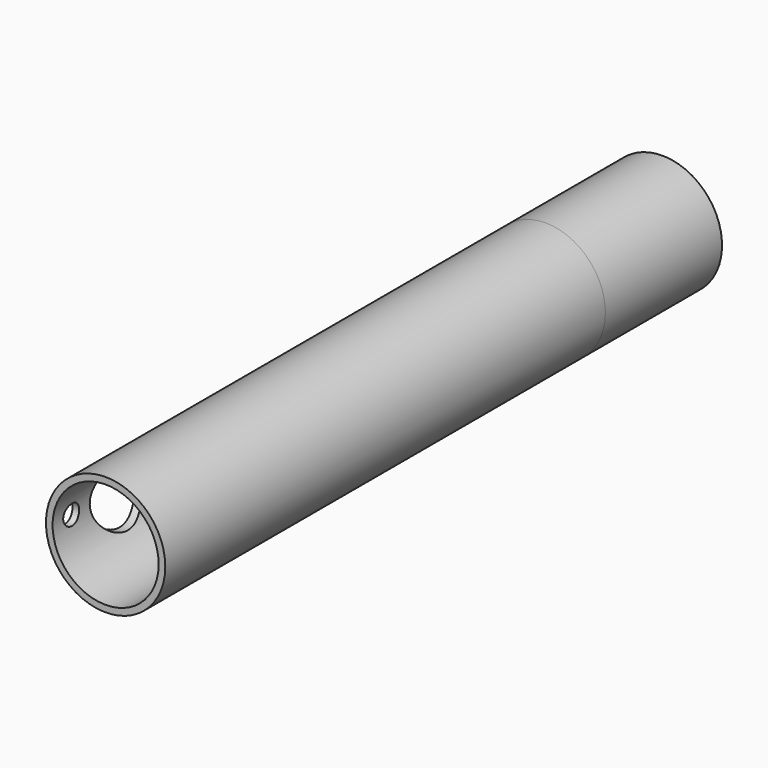
from build123d import *

# Parameters (mm, degrees)
F3_R      = 4.5
F4_DEPTH  = 32.5
F8_DEPTH  = 32.5
F6_R      = 4.5
F6_R_2    = 4
F9_DEPTH  = 9
F7_R      = 4.5
F7_R_2    = 4
F10_DEPTH = 11
F11_R     = 2.5
F11_R_2   = 0.75
F12_DEPTH = 4.501


# Not quite as in the source:
# - ends of sketch curves that miss each other by under 0.0002 mm in the source are joined


with BuildPart() as f4:
    # F3 (on Front) → F4 (new body)
    with BuildSketch(Plane.XZ):
        Circle(F3_R)
    extrude(amount=F4_DEPTH)

    # F5 (on face) → F8 (cut, through all)
    with BuildSketch(Plane.XZ.offset(32.5)):
        with BuildLine():
            Line((-1.25, -3.8), (0, -3.8))
            Line((0, -3.8), (1.25, -3.8))
            Line((1.25, -3.8), (1.25, -3.7))
            ThreePointArc((1.25, -3.7), (1.3085786438, -3.5585786438), (1.45, -3.5))
            Line((1.45, -3.5), (2, -3.5))
            Line((2, -3.5), (2, -3.05))
            ThreePointArc((2, -3.05), (2.0585786438, -2.9085786438), (2.2, -2.85))
            Line((2.2, -2.85), (3.15, -2.85))
            Line((3.15, -2.85), (3.15, -2.15))
            Line((3.15, -2.15), (2.2, -2.15))
            ThreePointArc((2.2, -2.15), (2.0585786438, -2.0914213562), (2, -1.95))
            Line((2, -1.95), (2, -1.887459))
            ThreePointArc((2, -1.887459), (2.1033535752, -1.771554046), (2.2, -1.65))
            Line((2.2, -1.65), (3.75, -1.65))
            Line((3.75, -1.65), (3.75, 0))
            Line((3.75, 0), (3.75, 1.65))
            Line((3.75, 1.65), (2.2, 1.65))
            ThreePointArc((2.2, 1.65), (2.1033535752, 1.771554046), (1.9999998047, 1.8874588157))
            Line((1.9999998047, 1.8874588157), (2, 1.95))
            ThreePointArc((2, 1.95), (2.0585786438, 2.0914213562), (2.2, 2.15))
            Line((2.2, 2.15), (3.15, 2.15))
            Line((3.15, 2.15), (3.15, 2.85))
            Line((3.15, 2.85), (2.2, 2.85))
            ThreePointArc((2.2, 2.85), (2.0585786438, 2.9085786438), (2, 3.05))
            Line((2, 3.05), (2, 3.5))
            Line((2, 3.5), (1.45, 3.5))
            ThreePointArc((1.45, 3.5), (1.3085786438, 3.5585786438), (1.25, 3.7))
            Line((1.25, 3.7), (1.25, 3.8))
            Line((1.25, 3.8), (0, 3.8))
            Line((0, 3.8), (-1.25, 3.8))
            Line((-1.25, 3.8), (-1.25, 3.7))
            ThreePointArc((-1.25, 3.7), (-1.3085786438, 3.5585786438), (-1.45, 3.5))
            Line((-1.45, 3.5), (-2, 3.5))
            Line((-2, 3.5), (-2, 3.05))
            ThreePointArc((-2, 3.05), (-2.0585786438, 2.9085786438), (-2.2, 2.85))
            Line((-2.2, 2.85), (-3.15, 2.85))
            Line((-3.15, 2.85), (-3.15, 2.15))
            Line((-3.15, 2.15), (-2.2, 2.15))
            ThreePointArc((-2.2, 2.15), (-2.0585786438, 2.0914213562), (-2, 1.95))
            Line((-2, 1.95), (-2, 1.887459))
            ThreePointArc((-2, 1.887459), (-2.1033535752, 1.771554046), (-2.2, 1.65))
            Line((-2.2, 1.65), (-3.75, 1.65))
            Line((-3.75, 1.65), (-3.75, 0))
            Line((-3.75, 0), (-3.75, -1.65))
            Line((-3.75, -1.65), (-2.2, -1.65))
            ThreePointArc((-2.2, -1.65), (-2.1033535752, -1.771554046), (-1.9999998047, -1.8874588157))
            Line((-1.9999998047, -1.8874588157), (-2, -1.95))
            ThreePointArc((-2, -1.95), (-2.0585786438, -2.0914213562), (-2.2, -2.15))
            Line((-2.2, -2.15), (-3.15, -2.15))
            Line((-3.15, -2.15), (-3.15, -2.85))
            Line((-3.15, -2.85), (-2.2, -2.85))
            ThreePointArc((-2.2, -2.85), (-2.0585786438, -2.9085786438), (-2, -3.05))
            Line((-2, -3.05), (-2, -3.5))
            Line((-2, -3.5), (-1.45, -3.5))
            ThreePointArc((-1.45, -3.5), (-1.3085786438, -3.5585786438), (-1.25, -3.7))
            Line((-1.25, -3.7), (-1.25, -3.8))
        make_face()
    extrude(amount=-F8_DEPTH, mode=Mode.SUBTRACT)

    # F6 (on face) → F9 (join)
    with BuildSketch(Plane.XZ.offset(32.5)):
        Circle(F6_R)
        Circle(F6_R_2, mode=Mode.SUBTRACT)
    extrude(amount=F9_DEPTH)

    # F7 (on face) → F10 (join)
    with BuildSketch(Plane(origin=(0, 0, 0), x_dir=(-1, 0, 0), z_dir=(0, 1, 0))):
        Circle(F7_R)
        Circle(F7_R_2, mode=Mode.SUBTRACT)
    extrude(amount=F10_DEPTH)

    # F11 (on Right) → F12 (cut, through all)
    with BuildSketch(Plane.YZ):
        with Locations((-35.5, 0)):
            Circle(F11_R)
        with Locations((-39.75, 0)):
            Circle(F11_R_2)
    extrude(amount=-F12_DEPTH, mode=Mode.SUBTRACT)


solid = f4.part
